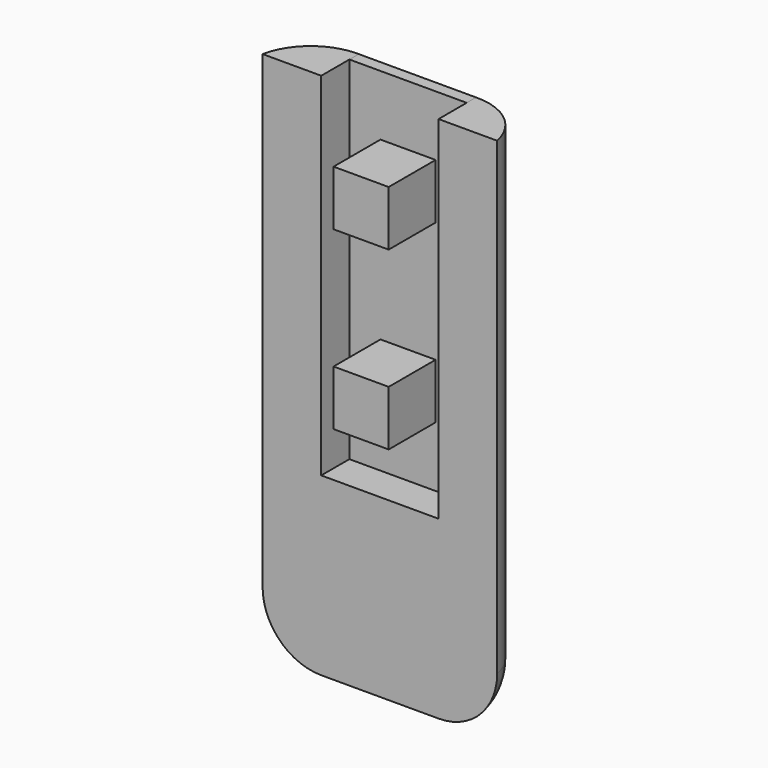
from build123d import *

# Parameters (mm, degrees)
F1_DEPTH    = 4
F2_T1_DEPTH = 52.2474487139
F2_T3_DEPTH = 10
F2_T6_ANGLE = 90
F2_T8_ANGLE = 90
F0_W        = 4.7
F0_H        = 4.7
F3_DEPTH    = 6
F0_W_2      = 10
F0_H_2      = 30
F4_DEPTH    = 1


# Not quite as in the source:
# - a fillet or chamfer that OpenCascade refuses, or shapes differently, is made with other operations: its cross-section is extruded or revolved along the edge and cut away or added


with BuildPart() as f1:
    # F0 (on Front) → F1 (new body)
    with BuildSketch(Plane.XZ):
        with BuildLine():
            ThreePointArc((-10, -17.5), (-8.5355339059, -21.0355339059), (-5, -22.5))
            Line((-5, -22.5), (5, -22.5))
            ThreePointArc((5, -22.5), (8.5355339059, -21.0355339059), (10, -17.5))
            Line((10, -17.5), (10, 22.5))
            Line((10, 22.5), (5, 22.5))
            Line((5, 22.5), (5, -7.5))
            Line((5, -7.5), (-5, -7.5))
            Line((-5, -7.5), (-5, 22.5))
            Line((-5, 22.5), (-10, 22.5))
            Line((-10, 22.5), (-10, -17.5))
        make_face()
    extrude(amount=F1_DEPTH)

    # F2: fillet of radius 5 on 1 edges, made by hand

    # F2_s2 → F2_t1 (cut)
    with BuildSketch(Plane.XY.offset(-17.5)):
        with BuildLine():
            ThreePointArc((10, -4), (8.2632981746, -1.1270166538), (5.1010205144, 0))
            Line((5.1010205144, 0), (10, 0))
            Line((10, 0), (10, -4))
        make_face()
        with BuildLine():
            ThreePointArc((-10, -4), (-8.2632981746, -1.1270166538), (-5.1010205144, 0))
            Line((-5.1010205144, 0), (-10, 0))
            Line((-10, 0), (-10, -4))
        make_face()
    extrude(amount=F2_T1_DEPTH, mode=Mode.SUBTRACT)

    # F2_s4 → F2_t3 (cut)
    with BuildSketch(Plane.YZ.offset(-5)):
        with BuildLine():
            ThreePointArc((-4, -22.5), (-1.1270166538, -20.7632981746), (0, -17.6010205144))
            Line((0, -17.6010205144), (0, -22.5))
            Line((0, -22.5), (-4, -22.5))
        make_face()
    extrude(amount=F2_T3_DEPTH, mode=Mode.SUBTRACT)

    # F2_s5 → F2_t6 (revolve, cut)
    with BuildSketch(Plane.YZ.offset(5)):
        with BuildLine():
            ThreePointArc((-4, -22.5), (-1.1270166538, -20.7632981746), (0, -17.6010205144))
            Line((0, -17.6010205144), (0, -22.5))
            Line((0, -22.5), (-4, -22.5))
        make_face()
    revolve(axis=Axis((5, 0, -17.5), (0, -1, 0)), revolution_arc=F2_T6_ANGLE, mode=Mode.SUBTRACT)

    # F2_s7 → F2_t8 (revolve, cut)
    with BuildSketch(Plane.XY.offset(-17.5)):
        with BuildLine():
            ThreePointArc((-10, -4), (-8.2632981746, -1.1270166538), (-5.1010205144, 0))
            Line((-5.1010205144, 0), (-10, 0))
            Line((-10, 0), (-10, -4))
        make_face()
    revolve(axis=Axis((-5, 0, -17.5), (0, -1, 0)), revolution_arc=F2_T8_ANGLE, mode=Mode.SUBTRACT)


with BuildPart() as f3:
    # F0 (on Front) → F3 (new body)
    with BuildSketch(Plane.XZ):
        Rectangle(F0_W, F0_H)
    extrude(amount=F3_DEPTH)


with BuildPart() as f3b:
    # F0 (on Front) → F3, piece 2 (new body)
    with BuildSketch(Plane.XZ):
        with Locations((0, 15)):
            Rectangle(F0_W, F0_H)
    extrude(amount=F3_DEPTH)


with BuildPart() as f4:
    # F0 (on Front) → F4 (new body)
    with BuildSketch(Plane.XZ):
        with Locations((0, 7.5)):
            Rectangle(F0_W_2, F0_H_2)
        Rectangle(F0_W, F0_H, mode=Mode.SUBTRACT)
        with Locations((0, 15)):
            Rectangle(F0_W, F0_H, mode=Mode.SUBTRACT)
    extrude(amount=F4_DEPTH)


solid = Compound([f1.part, f3.part, f3b.part, f4.part])
